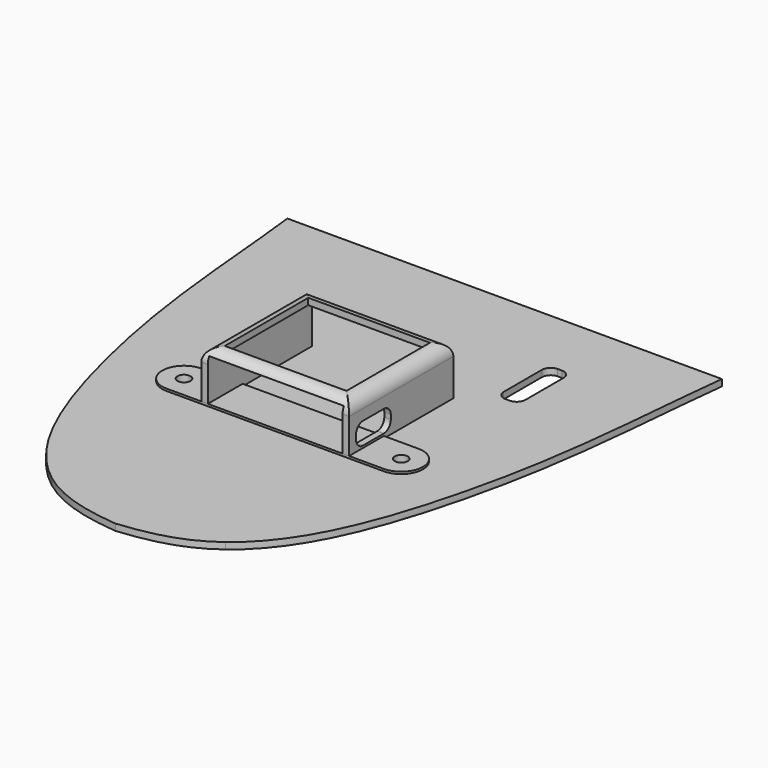
from build123d import *

# Parameters (mm, degrees)
F0_R        = 6
F0_W        = 5
F0_H        = 15
F0_R_2      = 3
F0_R_3      = 1.5
F1_DEPTH    = 1.5
F2_DEPTH    = 13
F3_T        = -1.5
F4_T1_DEPTH = 45
F4_T3_DEPTH = 49
F5_R        = 2
F6_DEPTH    = 2
F7_START    = 3
F7_DEPTH    = 22
F8_W        = 10
F8_H        = 5
F9_DEPTH    = 5
F10_R       = 2


# Not quite as in the source:
# - a fillet or chamfer that OpenCascade refuses, or shapes differently, is made with other operations: its cross-section is extruded or revolved along the edge and cut away or added


with BuildPart() as f1:
    # F0 (on Top) → F1 (new body)
    with BuildSketch(Plane.XY):
        with BuildLine():
            Line((50, 74.6730720997), (0, 74.6730720997))
            Line((0, 74.6730720997), (0, 69.6730720997))
            Line((0, 69.6730720997), (0, 64.6730720997))
            Line((0, 64.6730720997), (0, 38.6730720997))
            Line((0, 38.6730720997), (17, 38.6730720997))
            Line((17, 38.6730720997), (17, 18.6727328867))
            Line((17, 18.6727328867), (24.9997879891, 18.6730720952))
            ThreePointArc((24.9997879891, 18.6730720952), (28.535458948, 17.208680962), (30, 13.6730720997))
            ThreePointArc((30, 13.6730720997), (28.5355339059, 10.1375381938), (25, 8.6730720997))
            Line((25, 8.6730720997), (17, 8.6730720997))
            Line((17, 8.6730720997), (0, 8.6730720997))
            Line((0, 8.6730720997), (0, 7.6730720997))
            Line((0, 7.6730720997), (20, 7.6730720997))
            Line((20, 7.6730720997), (20, -1.4825001728))
            ThreePointArc((20, -1.4825001728), (23.3406734607, -3.5949503292), (24.642552197, -7.3269279003))
            ThreePointArc((24.642552197, -7.3269279003), (23.3406734607, -11.0589054714), (20, -13.1713556278))
            Line((20, -13.1713556278), (20, -30.6029154708))
            add(Edge.make_bspline(
                [(50, 74.6730720997), (49.0459845068, 66.9929651356), (47.3037907792, 43.380231158), (42.8042626578, 15.237762147), (33.9460152145, -15.0102641191), (24.7180314416, -27.0363946308), (20, -30.6029154708)],
                knots=[0, 0, 0, 0, 0.2142082733, 0.4293529985, 0.6487321082, 0.8142938826, 0.8142938826, 0.8142938826, 0.8142938826], degree=3))
        make_face()
        with Locations((29.4684451073, 27.5630913675)):
            Circle(F0_R, mode=Mode.SUBTRACT)
        with Locations((15, 61.6730720997)):
            Circle(F0_R, mode=Mode.SUBTRACT)
        with Locations((25, 51.7858859897)):
            Rectangle(F0_W, F0_H, mode=Mode.SUBTRACT)
        with Locations((35, 61.6730720997)):
            Circle(F0_R, mode=Mode.SUBTRACT)
        with BuildLine():
            Line((0, 69.6730720997), (0, 74.6730720997))
            Line((0, 74.6730720997), (-50, 74.6730720997))
            add(Edge.make_bspline(
                [(-50, 74.6730720997), (-49.0459845068, 66.9929651356), (-47.3037907792, 43.380231158), (-42.8042626578, 15.237762147), (-33.9460152145, -15.0102641191), (-24.7180314416, -27.0363946308), (-20, -30.6029154708)],
                knots=[0, 0, 0, 0, 0.2142082733, 0.4293529985, 0.6487321082, 0.8142938826, 0.8142938826, 0.8142938826, 0.8142938826], degree=3))
            Line((-20, -30.6029154708), (-20, -13.1713556278))
            ThreePointArc((-20, -13.1713556278), (-24.642552197, -7.3269279003), (-20, -1.4825001728))
            Line((-20, -1.4825001728), (-20, 7.6730720997))
            Line((-20, 7.6730720997), (0, 7.6730720997))
            Line((0, 7.6730720997), (0, 8.6730720997))
            Line((0, 8.6730720997), (-17, 8.6730720997))
            Line((-17, 8.6730720997), (-25, 8.6730720997))
            ThreePointArc((-25, 8.6730720997), (-29.999471487, 13.7457690764), (-24.854621415, 18.6709581595))
            Line((-24.854621415, 18.6709581595), (-17, 18.6712912126))
            Line((-17, 18.6712912126), (-17, 38.6730720997))
            Line((-17, 38.6730720997), (0, 38.6730720997))
            Line((0, 38.6730720997), (0, 64.6730720997))
            Line((0, 64.6730720997), (0, 69.6730720997))
        make_face()
        with Locations((-29.4684451073, 27.5630913675)):
            Circle(F0_R, mode=Mode.SUBTRACT)
        with Locations((-35, 61.6730720997)):
            Circle(F0_R, mode=Mode.SUBTRACT)
        with Locations((-25, 47.6730720997)):
            Circle(F0_R, mode=Mode.SUBTRACT)
        with Locations((-15, 61.6730720997)):
            Circle(F0_R, mode=Mode.SUBTRACT)
        with BuildLine():
            add(Edge.make_bspline(
                [(20, -30.6029154708), (19.6703346362, -30.85212076), (14.3195363247, -34.7267287684), (8.0180540099, -36.5596981444), (0, -37.3269279003)],
                knots=[0.8142938826, 0.8142938826, 0.8142938826, 0.8142938826, 0.825862263, 1, 1, 1, 1], degree=3))
            Line((20, -30.6029154708), (20, -13.1713556278))
            ThreePointArc((20, -13.1713556278), (12.642552197, -7.3269279003), (20, -1.4825001728))
            Line((20, -1.4825001728), (20, 7.6730720997))
            Line((20, 7.6730720997), (0, 7.6730720997))
            Line((0, 7.6730720997), (0, -1.3269279003))
            ThreePointArc((0, -1.3269279003), (4.2426406871, -3.0842872132), (6, -7.3269279003))
            ThreePointArc((6, -7.3269279003), (4.2426406871, -11.5695685874), (0, -13.3269279003))
            Line((0, -13.3269279003), (0, -21.1192360669))
            ThreePointArc((0, -21.1192360669), (4.2426406871, -22.8765953798), (6, -27.1192360669))
            ThreePointArc((6, -27.1192360669), (4.2426406871, -31.3618767541), (0, -33.1192360669))
            Line((0, -33.1192360669), (0, -37.3269279003))
        make_face()
        with BuildLine():
            Line((-20, -13.1713556278), (-20, -30.6029154708))
            add(Edge.make_bspline(
                [(-20, -30.6029154708), (-19.6703346362, -30.85212076), (-14.3195363247, -34.7267287684), (-8.0180540099, -36.5596981444), (0, -37.3269279003)],
                knots=[0.8142938826, 0.8142938826, 0.8142938826, 0.8142938826, 0.825862263, 1, 1, 1, 1], degree=3))
            Line((0, -37.3269279003), (0, -33.1192360669))
            ThreePointArc((0, -33.1192360669), (-6, -27.1192360669), (0, -21.1192360669))
            Line((0, -21.1192360669), (0, -13.3269279003))
            ThreePointArc((0, -13.3269279003), (-6, -7.3269279003), (0, -1.3269279003))
            Line((0, -1.3269279003), (0, 7.6730720997))
            Line((0, 7.6730720997), (-20, 7.6730720997))
            Line((-20, 7.6730720997), (-20, -1.4825001728))
            ThreePointArc((-20, -1.4825001728), (-14.9105746259, -2.6288066365), (-12.642552197, -7.3269279003))
            ThreePointArc((-12.642552197, -7.3269279003), (-14.9105746259, -12.0250491641), (-20, -13.1713556278))
        make_face()
        with BuildLine():
            ThreePointArc((20, -1.4825001728), (12.642552197, -7.3269279003), (20, -13.1713556278))
            Line((20, -13.1713556278), (20, -1.4825001728))
        make_face()
        with BuildLine():
            Line((20, -1.4825001728), (20, -13.1713556278))
            ThreePointArc((20, -13.1713556278), (23.3406734607, -11.0589054714), (24.642552197, -7.3269279003))
            ThreePointArc((24.642552197, -7.3269279003), (23.3406734607, -3.5949503292), (20, -1.4825001728))
        make_face()
        Polygon((17, 38.6730720997), (0, 38.6730720997), (0, 35.6730720997), (14, 35.6730720997), (14, 18.6726056802), (17, 18.6727328867), align=None)
        Polygon((0, 35.6730720997), (0, 38.6730720997), (-17, 38.6730720997), (-17, 18.6712912126), (-14, 18.6714184191), (-14, 35.6730720997), align=None)
        with BuildLine():
            ThreePointArc((-20, -1.4825001728), (-24.642552197, -7.3269279003), (-20, -13.1713556278))
            Line((-20, -13.1713556278), (-20, -1.4825001728))
        make_face()
        with BuildLine():
            Line((-20, -1.4825001728), (-20, -13.1713556278))
            ThreePointArc((-20, -13.1713556278), (-14.9105746259, -12.0250491641), (-12.642552197, -7.3269279003))
            ThreePointArc((-12.642552197, -7.3269279003), (-14.9105746259, -2.6288066365), (-20, -1.4825001728))
        make_face()
        with BuildLine():
            ThreePointArc((0, -21.1192360669), (-6, -27.1192360669), (0, -33.1192360669))
            Line((0, -33.1192360669), (0, -21.1192360669))
        make_face()
        with BuildLine():
            Line((0, -21.1192360669), (0, -33.1192360669))
            ThreePointArc((0, -33.1192360669), (4.2426406871, -31.3618767541), (6, -27.1192360669))
            ThreePointArc((6, -27.1192360669), (4.2426406871, -22.8765953798), (0, -21.1192360669))
        make_face()
        Polygon((14, 35.6730720997), (0, 35.6730720997), (0, 18.6720120497), (14, 18.6726056802), align=None)
        Polygon((0, 18.6720120497), (0, 35.6730720997), (-14, 35.6730720997), (-14, 18.6714184191), align=None)
        Polygon((14, 18.6726056802), (0, 18.6720120497), (0, 11.6730720997), (14, 11.6730720997), align=None)
        Polygon((0, 11.6730720997), (0, 18.6720120497), (-14, 18.6714184191), (-14, 11.6730720997), align=None)
        with BuildLine():
            Line((24.9997879891, 18.6730720952), (17, 18.6727328867))
            Line((17, 18.6727328867), (17, 8.6730720997))
            Line((17, 8.6730720997), (25, 8.6730720997))
            ThreePointArc((25, 8.6730720997), (20.0000000011, 13.6729660942), (24.9997879891, 18.6730720952))
        make_face()
        Polygon((17, 8.6730720997), (17, 18.6727328867), (14, 18.6726056802), (14, 11.6730720997), (0, 11.6730720997), (0, 8.6730720997), align=None)
        Polygon((-14, 18.6714184191), (-17, 18.6712912126), (-17, 8.6730720997), (0, 8.6730720997), (0, 11.6730720997), (-14, 11.6730720997), align=None)
        with BuildLine():
            Line((-17, 8.6730720997), (-17, 18.6712912126))
            Line((-17, 18.6712912126), (-24.854621415, 18.6709581595))
            ThreePointArc((-24.854621415, 18.6709581595), (-21.4134352839, 17.1568277653), (-20, 13.6730720997))
            ThreePointArc((-20, 13.6730720997), (-21.4644660941, 10.1375381938), (-25, 8.6730720997))
            Line((-25, 8.6730720997), (-17, 8.6730720997))
        make_face()
        with BuildLine():
            ThreePointArc((0, -1.3269279003), (-6, -7.3269279003), (0, -13.3269279003))
            Line((0, -13.3269279003), (0, -1.3269279003))
        make_face()
        with BuildLine():
            Line((0, -1.3269279003), (0, -13.3269279003))
            ThreePointArc((0, -13.3269279003), (4.2426406871, -11.5695685874), (6, -7.3269279003))
            ThreePointArc((6, -7.3269279003), (4.2426406871, -3.0842872132), (0, -1.3269279003))
        make_face()
        with BuildLine():
            ThreePointArc((30, 13.6730720997), (28.535458948, 17.208680962), (24.9997879891, 18.6730720952))
            ThreePointArc((24.9997879891, 18.6730720952), (20.0000000011, 13.6729660942), (25, 8.6730720997))
            ThreePointArc((25, 8.6730720997), (28.5355339059, 10.1375381938), (30, 13.6730720997))
        make_face()
        with Locations((25, 13.6730720997)):
            Circle(F0_R_2, mode=Mode.SUBTRACT)
        with BuildLine():
            ThreePointArc((-20, 13.6730720997), (-21.4134352839, 17.1568277653), (-24.854621415, 18.6709581595))
            ThreePointArc((-24.854621415, 18.6709581595), (-29.999471487, 13.7457690764), (-25, 8.6730720997))
            ThreePointArc((-25, 8.6730720997), (-21.4644660941, 10.1375381938), (-20, 13.6730720997))
        make_face()
        with Locations((-25, 13.6730720997)):
            Circle(F0_R_2, mode=Mode.SUBTRACT)
        with Locations((-25, 13.6730720997)):
            Circle(F0_R_2)
        with Locations((-25, 13.6730720997)):
            Circle(F0_R_3, mode=Mode.SUBTRACT)
        with Locations((25, 13.6730720997)):
            Circle(F0_R_2)
        with Locations((25, 13.6730720997)):
            Circle(F0_R_3, mode=Mode.SUBTRACT)
        with Locations((-35, 61.6730720997)):
            Circle(F0_R)
        with Locations((-15, 61.6730720997)):
            Circle(F0_R)
        with Locations((-25, 47.6730720997)):
            Circle(F0_R)
        with Locations((-29.4684451073, 27.5630913675)):
            Circle(F0_R)
        with Locations((35, 61.6730720997)):
            Circle(F0_R)
        with Locations((29.4684451073, 27.5630913675)):
            Circle(F0_R)
        with Locations((15, 61.6730720997)):
            Circle(F0_R)
    extrude(amount=F1_DEPTH)

    # F0 (on Top) → F2 (join)
    with BuildSketch(Plane.XY):
        Polygon((0, 18.6720120497), (0, 35.6730720997), (-14, 35.6730720997), (-14, 18.6714184191), align=None)
        Polygon((14, 35.6730720997), (0, 35.6730720997), (0, 18.6720120497), (14, 18.6726056802), align=None)
        Polygon((14, 18.6726056802), (0, 18.6720120497), (0, 11.6730720997), (14, 11.6730720997), align=None)
        Polygon((0, 11.6730720997), (0, 18.6720120497), (-14, 18.6714184191), (-14, 11.6730720997), align=None)
        Polygon((0, 35.6730720997), (0, 38.6730720997), (-17, 38.6730720997), (-17, 18.6712912126), (-14, 18.6714184191), (-14, 35.6730720997), align=None)
        Polygon((17, 38.6730720997), (0, 38.6730720997), (0, 35.6730720997), (14, 35.6730720997), (14, 18.6726056802), (17, 18.6727328867), align=None)
        Polygon((17, 8.6730720997), (17, 18.6727328867), (14, 18.6726056802), (14, 11.6730720997), (0, 11.6730720997), (0, 8.6730720997), align=None)
        Polygon((-14, 18.6714184191), (-17, 18.6712912126), (-17, 8.6730720997), (0, 8.6730720997), (0, 11.6730720997), (-14, 11.6730720997), align=None)
    extrude(amount=F2_DEPTH)

    # F3: a shell. OpenCascade refuses it in one call, so the cavity is built on its own and cut out:
    # the body offset inwards by the wall thickness, plus a prism from it out through each open face.
    f3_core = offset(f1.part, amount=F3_T, kind=Kind.INTERSECTION, mode=Mode.PRIVATE)
    f3_exits = [f3_core.faces().sort_by_distance(p)[0] for p in [
        (0, 10.173072, 6.5),
        (0, 37.173072, 6.5),
    ]]
    add(f3_core, mode=Mode.SUBTRACT)
    extrude(f3_exits, amount=-F3_T, mode=Mode.SUBTRACT)

    # F4: fillet of radius 3 on 4 edges, made by hand

    # F4_s2 → F4_t1 (cut)
    with BuildSketch(Plane.XZ.offset(-46.1730720997)):
        with BuildLine():
            ThreePointArc((-14, 13), (-16.1213203436, 12.1213203436), (-17, 10))
            Line((-17, 10), (-17, 13))
            Line((-17, 13), (-14, 13))
        make_face()
        with BuildLine():
            ThreePointArc((17, 10), (16.1213203436, 12.1213203436), (14, 13))
            Line((14, 13), (17, 13))
            Line((17, 13), (17, 10))
        make_face()
    extrude(amount=F4_T1_DEPTH, mode=Mode.SUBTRACT)

    # F4_s4 → F4_t3 (cut)
    with BuildSketch(Plane.YZ.offset(-24.5)):
        with BuildLine():
            ThreePointArc((11.6730720997, 13), (9.5517517561, 12.1213203436), (8.6730720997, 10))
            Line((8.6730720997, 10), (8.6730720997, 13))
            Line((8.6730720997, 13), (11.6730720997, 13))
        make_face()
        with BuildLine():
            ThreePointArc((35.6730720997, 13), (37.7943924432, 12.1213203436), (38.6730720997, 10))
            Line((38.6730720997, 10), (38.6730720997, 13))
            Line((38.6730720997, 13), (35.6730720997, 13))
        make_face()
    extrude(amount=F4_T3_DEPTH, mode=Mode.SUBTRACT)

    # F5
    f5_edges = [f1.edges().sort_by_distance(p)[0] for p in [
        (22.5, 59.285886, 0.75),
        (27.5, 59.285886, 0.75),
        (27.5, 44.285886, 0.75),
        (22.5, 44.285886, 0.75),
    ]]
    fillet(f5_edges, radius=F5_R)

    # F0 (on Top) → F7 (cut)
    with BuildSketch(Plane.XY.offset(F7_START)):
        Polygon((0, 18.6720120497), (0, 35.6730720997), (-14, 35.6730720997), (-14, 18.6714184191), align=None)
        Polygon((14, 35.6730720997), (0, 35.6730720997), (0, 18.6720120497), (14, 18.6726056802), align=None)
        Polygon((14, 18.6726056802), (0, 18.6720120497), (0, 11.6730720997), (14, 11.6730720997), align=None)
        Polygon((0, 11.6730720997), (0, 18.6720120497), (-14, 18.6714184191), (-14, 11.6730720997), align=None)
    extrude(amount=F7_DEPTH, mode=Mode.SUBTRACT)

    # F8 (on face) → F9 (cut)
    with BuildSketch(Plane.YZ.offset(17)):
        with Locations((15.6730720997, 5)):
            Rectangle(F8_W, F8_H)
    extrude(amount=-F9_DEPTH, mode=Mode.SUBTRACT)

    # F10
    f10_edges = [f1.edges().sort_by_distance(p)[0] for p in [
        (16.25, 20.673072, 2.5),
        (16.25, 20.673072, 7.5),
        (16.25, 10.673072, 7.5),
        (16.25, 10.673072, 2.5),
    ]]
    fillet(f10_edges, radius=F10_R)


with BuildPart() as f6:
    # F0 (on Top) → F6 (new body)
    with BuildSketch(Plane.XY):
        Polygon((14, 18.6726056802), (0, 18.6720120497), (0, 11.6730720997), (14, 11.6730720997), align=None)
        Polygon((0, 11.6730720997), (0, 18.6720120497), (-14, 18.6714184191), (-14, 11.6730720997), align=None)
        with BuildLine():
            Line((24.9997879891, 18.6730720952), (17, 18.6727328867))
            Line((17, 18.6727328867), (17, 8.6730720997))
            Line((17, 8.6730720997), (25, 8.6730720997))
            ThreePointArc((25, 8.6730720997), (20.0000000011, 13.6729660942), (24.9997879891, 18.6730720952))
        make_face()
        Polygon((17, 8.6730720997), (17, 18.6727328867), (14, 18.6726056802), (14, 11.6730720997), (0, 11.6730720997), (0, 8.6730720997), align=None)
        Polygon((-14, 18.6714184191), (-17, 18.6712912126), (-17, 8.6730720997), (0, 8.6730720997), (0, 11.6730720997), (-14, 11.6730720997), align=None)
        with BuildLine():
            Line((-17, 8.6730720997), (-17, 18.6712912126))
            Line((-17, 18.6712912126), (-24.854621415, 18.6709581595))
            ThreePointArc((-24.854621415, 18.6709581595), (-21.4134352839, 17.1568277653), (-20, 13.6730720997))
            ThreePointArc((-20, 13.6730720997), (-21.4644660941, 10.1375381938), (-25, 8.6730720997))
            Line((-25, 8.6730720997), (-17, 8.6730720997))
        make_face()
        with BuildLine():
            ThreePointArc((30, 13.6730720997), (28.535458948, 17.208680962), (24.9997879891, 18.6730720952))
            ThreePointArc((24.9997879891, 18.6730720952), (20.0000000011, 13.6729660942), (25, 8.6730720997))
            ThreePointArc((25, 8.6730720997), (28.5355339059, 10.1375381938), (30, 13.6730720997))
        make_face()
        with Locations((25, 13.6730720997)):
            Circle(F0_R_2, mode=Mode.SUBTRACT)
        with BuildLine():
            ThreePointArc((-20, 13.6730720997), (-21.4134352839, 17.1568277653), (-24.854621415, 18.6709581595))
            ThreePointArc((-24.854621415, 18.6709581595), (-29.999471487, 13.7457690764), (-25, 8.6730720997))
            ThreePointArc((-25, 8.6730720997), (-21.4644660941, 10.1375381938), (-20, 13.6730720997))
        make_face()
        with Locations((-25, 13.6730720997)):
            Circle(F0_R_2, mode=Mode.SUBTRACT)
        with Locations((-25, 13.6730720997)):
            Circle(F0_R_2)
        with Locations((-25, 13.6730720997)):
            Circle(F0_R_3, mode=Mode.SUBTRACT)
        with Locations((25, 13.6730720997)):
            Circle(F0_R_2)
        with Locations((25, 13.6730720997)):
            Circle(F0_R_3, mode=Mode.SUBTRACT)
    extrude(amount=F6_DEPTH)


solid = Compound([f1.part, f6.part])
